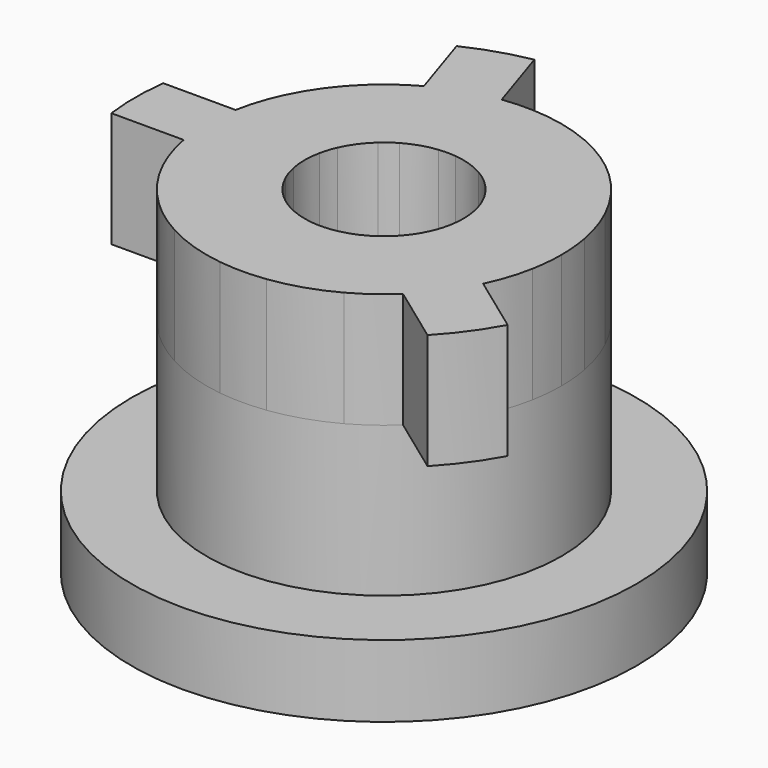
from build123d import *

# Parameters (mm, degrees)
F0_R     = 17.5
F0_R_2   = 5.5
F1_DEPTH = 5
F2_R     = 12.3
F2_R_2   = 5.5
F3_DEPTH = 10.4
F5_DEPTH = 8


with BuildPart() as f1:
    # F0 (on Top) → F1 (new body)
    with BuildSketch(Plane.XY):
        Circle(F0_R)
        Circle(F0_R_2, mode=Mode.SUBTRACT)
    extrude(amount=F1_DEPTH)

    # F2 (on face) → F3 (join)
    with BuildSketch(Plane.XY.offset(5)):
        Circle(F2_R)
        Circle(F2_R_2, mode=Mode.SUBTRACT)
    extrude(amount=F3_DEPTH)

    # F4 (on face) → F5 (join)
    with BuildSketch(Plane.XY.offset(15.4)):
        with BuildLine():
            Line((-1.5968973469, 12.1958976243), (-3.1451265822, 16.9608572537))
            ThreePointArc((-3.1451265822, 16.9608572537), (-5.330543153, 16.4057249061), (-7.4248809055, 15.5702807791))
            Line((-7.4248809055, 15.5702807791), (-5.8766516702, 10.8053211497))
            ThreePointArc((-5.8766516702, 10.8053211497), (-3.8009090308, 11.6979951504), (-1.5968973469, 12.1958976243))
        make_face()
        with BuildLine():
            ThreePointArc((-17.1026313765, 2.25), (-17.25, 0), (-17.1026313765, -2.25))
            Line((-17.1026313765, -2.25), (-12.0924563262, -2.25))
            ThreePointArc((-12.0924563262, -2.25), (-12.3, 0), (-12.0924563262, 2.25))
            Line((-12.0924563262, 2.25), (-17.1026313765, 2.25))
        make_face()
        with BuildLine():
            ThreePointArc((12.5138026145, -11.8729627358), (13.955543153, -10.139295602), (15.1588362498, -8.2323862612))
            Line((15.1588362498, -8.2323862612), (11.1055194893, -5.2874792552))
            ThreePointArc((11.1055194893, -5.2874792552), (9.9509090308, -7.2297586032), (8.4604858539, -8.9280557298))
            Line((8.4604858539, -8.9280557298), (12.5138026145, -11.8729627358))
        make_face()
        with BuildLine():
            Line((11.1055194893, -5.2874792552), (6.9247879586, -2.25))
            Line((6.9247879586, -2.25), (5.018714975, -2.25))
            ThreePointArc((5.018714975, -2.25), (4.4495934691, -3.2328188876), (3.6907453789, -4.077793343))
            Line((3.6907453789, -4.077793343), (4.2797543233, -5.8905764747))
            Line((4.2797543233, -5.8905764747), (8.4604858539, -8.9280557298))
            ThreePointArc((8.4604858539, -8.9280557298), (9.9509090308, -7.2297586032), (11.1055194893, -5.2874792552))
        make_face()
        with BuildLine():
            ThreePointArc((11.1055194893, -5.2874792552), (11.6979951504, -3.8009090308), (12.0924563262, -2.25))
            Line((12.0924563262, -2.25), (6.9247879586, -2.25))
            Line((6.9247879586, -2.25), (11.1055194893, -5.2874792552))
        make_face()
        with BuildLine():
            Line((6.9247879586, -2.25), (12.0924563262, -2.25))
            ThreePointArc((12.0924563262, -2.25), (12.2480041805, -1.1297759044), (12.3, 0))
            ThreePointArc((12.3, 0), (12.2480041805, 1.1297759044), (12.0924563262, 2.25))
            Line((12.0924563262, 2.25), (6.9247879586, 2.25))
            Line((6.9247879586, 2.25), (5.3827425223, 1.1296384104))
            ThreePointArc((5.3827425223, 1.1296384104), (5.4706070903, 0.5678539104), (5.5, 0))
            ThreePointArc((5.5, 0), (5.4706070903, -0.5678539104), (5.3827425223, -1.1296384104))
            Line((5.3827425223, -1.1296384104), (6.9247879586, -2.25))
        make_face()
        with BuildLine():
            Line((6.9247879586, 2.25), (12.0924563262, 2.25))
            ThreePointArc((12.0924563262, 2.25), (11.6979951504, 3.8009090308), (11.1055194893, 5.2874792552))
            Line((11.1055194893, 5.2874792552), (6.9247879586, 2.25))
        make_face()
        with BuildLine():
            Line((5.018714975, 2.25), (6.9247879586, 2.25))
            Line((6.9247879586, 2.25), (11.1055194893, 5.2874792552))
            ThreePointArc((11.1055194893, 5.2874792552), (9.9509090308, 7.2297586032), (8.4604858539, 8.9280557298))
            Line((8.4604858539, 8.9280557298), (4.2797543233, 5.8905764747))
            Line((4.2797543233, 5.8905764747), (3.6907453789, 4.077793343))
            ThreePointArc((3.6907453789, 4.077793343), (4.4495934691, 3.2328188876), (5.018714975, 2.25))
        make_face()
        with BuildLine():
            Line((4.2797543233, 5.8905764747), (8.4604858539, 8.9280557298))
            ThreePointArc((8.4604858539, 8.9280557298), (7.2297586032, 9.9509090308), (5.8766516702, 10.8053211497))
            Line((5.8766516702, 10.8053211497), (4.2797543233, 5.8905764747))
        make_face()
        with BuildLine():
            Line((2.737708887, 4.7702148851), (4.2797543233, 5.8905764747))
            Line((4.2797543233, 5.8905764747), (5.8766516702, 10.8053211497))
            ThreePointArc((5.8766516702, 10.8053211497), (3.8009090308, 11.6979951504), (1.5968973469, 12.1958976243))
            Line((1.5968973469, 12.1958976243), (0, 7.2811529494))
            Line((0, 7.2811529494), (0.5890089445, 5.4683698177))
            ThreePointArc((0.5890089445, 5.4683698177), (1.6995934691, 5.2308108396), (2.737708887, 4.7702148851))
        make_face()
        with BuildLine():
            Line((0, 7.2811529494), (1.5968973469, 12.1958976243))
            ThreePointArc((1.5968973469, 12.1958976243), (0, 12.3), (-1.5968973469, 12.1958976243))
            Line((-1.5968973469, 12.1958976243), (0, 7.2811529494))
        make_face()
        with BuildLine():
            Line((-0.5890089445, 5.4683698177), (0, 7.2811529494))
            Line((0, 7.2811529494), (-1.5968973469, 12.1958976243))
            ThreePointArc((-1.5968973469, 12.1958976243), (-3.8009090308, 11.6979951504), (-5.8766516702, 10.8053211497))
            Line((-5.8766516702, 10.8053211497), (-4.2797543233, 5.8905764747))
            Line((-4.2797543233, 5.8905764747), (-2.737708887, 4.7702148851))
            ThreePointArc((-2.737708887, 4.7702148851), (-1.6995934691, 5.2308108396), (-0.5890089445, 5.4683698177))
        make_face()
        with BuildLine():
            Line((-4.2797543233, 5.8905764747), (-5.8766516702, 10.8053211497))
            ThreePointArc((-5.8766516702, 10.8053211497), (-7.2297586032, 9.9509090308), (-8.4604858539, 8.9280557298))
            Line((-8.4604858539, 8.9280557298), (-4.2797543233, 5.8905764747))
        make_face()
        with BuildLine():
            Line((-3.6907453789, 4.077793343), (-4.2797543233, 5.8905764747))
            Line((-4.2797543233, 5.8905764747), (-8.4604858539, 8.9280557298))
            ThreePointArc((-8.4604858539, 8.9280557298), (-9.9509090308, 7.2297586032), (-11.1055194893, 5.2874792552))
            Line((-11.1055194893, 5.2874792552), (-6.9247879586, 2.25))
            Line((-6.9247879586, 2.25), (-5.018714975, 2.25))
            ThreePointArc((-5.018714975, 2.25), (-4.4495934691, 3.2328188876), (-3.6907453789, 4.077793343))
        make_face()
        with BuildLine():
            Line((-6.9247879586, 2.25), (-11.1055194893, 5.2874792552))
            ThreePointArc((-11.1055194893, 5.2874792552), (-11.6979951504, 3.8009090308), (-12.0924563262, 2.25))
            Line((-12.0924563262, 2.25), (-6.9247879586, 2.25))
        make_face()
        with BuildLine():
            Line((-12.0924563262, -2.25), (-6.9247879586, -2.25))
            Line((-6.9247879586, -2.25), (-5.3827425223, -1.1296384104))
            ThreePointArc((-5.3827425223, -1.1296384104), (-5.5, 0), (-5.3827425223, 1.1296384104))
            Line((-5.3827425223, 1.1296384104), (-6.9247879586, 2.25))
            Line((-6.9247879586, 2.25), (-12.0924563262, 2.25))
            ThreePointArc((-12.0924563262, 2.25), (-12.3, 0), (-12.0924563262, -2.25))
        make_face()
        with BuildLine():
            ThreePointArc((-12.0924563262, -2.25), (-11.6979951504, -3.8009090308), (-11.1055194893, -5.2874792552))
            Line((-11.1055194893, -5.2874792552), (-6.9247879586, -2.25))
            Line((-6.9247879586, -2.25), (-12.0924563262, -2.25))
        make_face()
        with BuildLine():
            Line((-8.4604858539, -8.9280557298), (-4.2797543233, -5.8905764747))
            Line((-4.2797543233, -5.8905764747), (-3.6907453789, -4.077793343))
            ThreePointArc((-3.6907453789, -4.077793343), (-4.4495934691, -3.2328188876), (-5.018714975, -2.25))
            Line((-5.018714975, -2.25), (-6.9247879586, -2.25))
            Line((-6.9247879586, -2.25), (-11.1055194893, -5.2874792552))
            ThreePointArc((-11.1055194893, -5.2874792552), (-9.9509090308, -7.2297586032), (-8.4604858539, -8.9280557298))
        make_face()
        with BuildLine():
            ThreePointArc((-8.4604858539, -8.9280557298), (-7.2297586032, -9.9509090308), (-5.8766516702, -10.8053211497))
            Line((-5.8766516702, -10.8053211497), (-4.2797543233, -5.8905764747))
            Line((-4.2797543233, -5.8905764747), (-8.4604858539, -8.9280557298))
        make_face()
        with BuildLine():
            Line((-1.5968973469, -12.1958976243), (0, -7.2811529494))
            Line((0, -7.2811529494), (-0.5890089445, -5.4683698177))
            ThreePointArc((-0.5890089445, -5.4683698177), (-1.6995934691, -5.2308108396), (-2.737708887, -4.7702148851))
            Line((-2.737708887, -4.7702148851), (-4.2797543233, -5.8905764747))
            Line((-4.2797543233, -5.8905764747), (-5.8766516702, -10.8053211497))
            ThreePointArc((-5.8766516702, -10.8053211497), (-3.8009090308, -11.6979951504), (-1.5968973469, -12.1958976243))
        make_face()
        with BuildLine():
            ThreePointArc((-1.5968973469, -12.1958976243), (0, -12.3), (1.5968973469, -12.1958976243))
            Line((1.5968973469, -12.1958976243), (0, -7.2811529494))
            Line((0, -7.2811529494), (-1.5968973469, -12.1958976243))
        make_face()
        with BuildLine():
            Line((5.8766516702, -10.8053211497), (4.2797543233, -5.8905764747))
            Line((4.2797543233, -5.8905764747), (2.737708887, -4.7702148851))
            ThreePointArc((2.737708887, -4.7702148851), (1.6995934691, -5.2308108396), (0.5890089445, -5.4683698177))
            Line((0.5890089445, -5.4683698177), (0, -7.2811529494))
            Line((0, -7.2811529494), (1.5968973469, -12.1958976243))
            ThreePointArc((1.5968973469, -12.1958976243), (3.8009090308, -11.6979951504), (5.8766516702, -10.8053211497))
        make_face()
        with BuildLine():
            ThreePointArc((5.8766516702, -10.8053211497), (7.2297586032, -9.9509090308), (8.4604858539, -8.9280557298))
            Line((8.4604858539, -8.9280557298), (4.2797543233, -5.8905764747))
            Line((4.2797543233, -5.8905764747), (5.8766516702, -10.8053211497))
        make_face()
        with BuildLine():
            Line((4.2797543233, -5.8905764747), (3.6907453789, -4.077793343))
            ThreePointArc((3.6907453789, -4.077793343), (3.2328188876, -4.4495934691), (2.737708887, -4.7702148851))
            Line((2.737708887, -4.7702148851), (4.2797543233, -5.8905764747))
        make_face()
        with BuildLine():
            Line((5.018714975, -2.25), (6.9247879586, -2.25))
            Line((6.9247879586, -2.25), (5.3827425223, -1.1296384104))
            ThreePointArc((5.3827425223, -1.1296384104), (5.2308108396, -1.6995934691), (5.018714975, -2.25))
        make_face()
        with BuildLine():
            Line((5.3827425223, 1.1296384104), (6.9247879586, 2.25))
            Line((6.9247879586, 2.25), (5.018714975, 2.25))
            ThreePointArc((5.018714975, 2.25), (5.2308108396, 1.6995934691), (5.3827425223, 1.1296384104))
        make_face()
        with BuildLine():
            ThreePointArc((2.737708887, 4.7702148851), (3.2328188876, 4.4495934691), (3.6907453789, 4.077793343))
            Line((3.6907453789, 4.077793343), (4.2797543233, 5.8905764747))
            Line((4.2797543233, 5.8905764747), (2.737708887, 4.7702148851))
        make_face()
        with BuildLine():
            ThreePointArc((-0.5890089445, 5.4683698177), (0, 5.5), (0.5890089445, 5.4683698177))
            Line((0.5890089445, 5.4683698177), (0, 7.2811529494))
            Line((0, 7.2811529494), (-0.5890089445, 5.4683698177))
        make_face()
        with BuildLine():
            ThreePointArc((-3.6907453789, 4.077793343), (-3.2328188876, 4.4495934691), (-2.737708887, 4.7702148851))
            Line((-2.737708887, 4.7702148851), (-4.2797543233, 5.8905764747))
            Line((-4.2797543233, 5.8905764747), (-3.6907453789, 4.077793343))
        make_face()
        with BuildLine():
            Line((-6.9247879586, 2.25), (-5.3827425223, 1.1296384104))
            ThreePointArc((-5.3827425223, 1.1296384104), (-5.2308108396, 1.6995934691), (-5.018714975, 2.25))
            Line((-5.018714975, 2.25), (-6.9247879586, 2.25))
        make_face()
        with BuildLine():
            Line((-6.9247879586, -2.25), (-5.018714975, -2.25))
            ThreePointArc((-5.018714975, -2.25), (-5.2308108396, -1.6995934691), (-5.3827425223, -1.1296384104))
            Line((-5.3827425223, -1.1296384104), (-6.9247879586, -2.25))
        make_face()
        with BuildLine():
            Line((-4.2797543233, -5.8905764747), (-2.737708887, -4.7702148851))
            ThreePointArc((-2.737708887, -4.7702148851), (-3.2328188876, -4.4495934691), (-3.6907453789, -4.077793343))
            Line((-3.6907453789, -4.077793343), (-4.2797543233, -5.8905764747))
        make_face()
        with BuildLine():
            Line((0, -7.2811529494), (0.5890089445, -5.4683698177))
            ThreePointArc((0.5890089445, -5.4683698177), (0, -5.5), (-0.5890089445, -5.4683698177))
            Line((-0.5890089445, -5.4683698177), (0, -7.2811529494))
        make_face()
    extrude(amount=F5_DEPTH)


solid = f1.part
